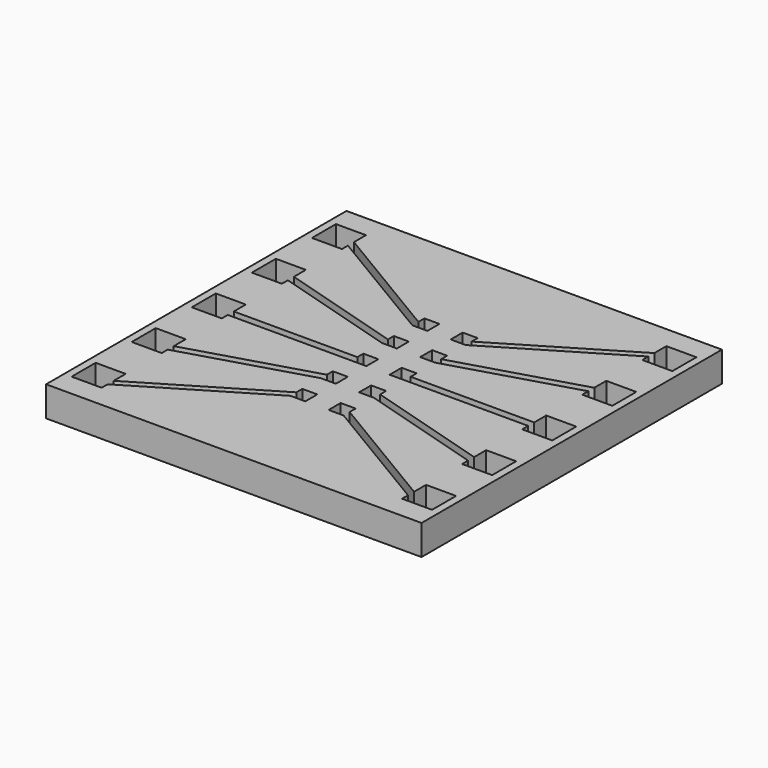
from build123d import *

# Parameters (mm, degrees)
F0_W     = 25
F0_H     = 25
F1_DEPTH = 2
F3_DEPTH = 2


# Not quite as in the source:
# - a feature names something its author has since deleted; it is built from what else it names


with BuildPart() as f1:
    # F0 (on Top) → F1 (new body)
    with BuildSketch(Plane.XY):
        with Locations((-12.5, 12.5)):
            Rectangle(F0_W, F0_H)
    extrude(amount=F1_DEPTH)

    # F2 (on face) → F3 (cut)
    with BuildSketch(Plane.XY.offset(2)):
        Polygon((-13.275, 15.54), (-14.275, 15.54), (-14.275, 15.04), (-22.5, 17.5), (-22.5, 18.5), (-24.5, 18.5), (-24.5, 16.5), (-22.5, 16.5), (-22.5, 17), (-14.275, 14.54), (-13.275, 14.54), align=None)
        Polygon((-13.275, 18.08), (-14.275, 18.08), (-14.275, 17.58), (-22.5, 22.5), (-22.5, 23.5), (-24.5, 23.5), (-24.5, 21.5), (-22.5, 21.5), (-22.5, 22), (-14.275, 17.08), (-13.275, 17.08), align=None)
        Polygon((-13.275, 13), (-14.275, 13), (-14.275, 12.5), (-22.5, 12.5), (-22.5, 13.5), (-24.5, 13.5), (-24.5, 11.5), (-22.5, 11.5), (-22.5, 12), (-14.275, 12), (-13.275, 12), align=None)
        Polygon((-13.275, 10.46), (-14.275, 10.46), (-14.275, 9.96), (-22.5, 7.5), (-22.5, 8.5), (-24.5, 8.5), (-24.5, 6.5), (-22.5, 6.5), (-22.5, 7), (-14.275, 9.46), (-13.275, 9.46), align=None)
        Polygon((-13.275, 7.92), (-14.275, 7.92), (-14.275, 7.42), (-22.5, 2.5), (-22.5, 3.5), (-24.5, 3.5), (-24.5, 1.5), (-22.5, 1.5), (-22.5, 2), (-14.275, 6.92), (-13.275, 6.92), align=None)
        Polygon((-10.725, 6.92), (-2.5, 2), (-2.5, 1.5), (-0.5, 1.5), (-0.5, 3.5), (-2.5, 3.5), (-2.5, 2.5), (-10.725, 7.42), (-10.725, 7.92), (-11.725, 7.92), (-11.725, 6.92), align=None)
        Polygon((-11.725, 12), (-10.725, 12), (-2.5, 12), (-2.5, 11.5), (-0.5, 11.5), (-0.5, 13.5), (-2.5, 13.5), (-2.5, 12.5), (-10.725, 12.5), (-10.725, 13), (-11.725, 13), align=None)
        Polygon((-11.725, 14.54), (-10.725, 14.54), (-2.5, 17), (-2.5, 16.5), (-0.5, 16.5), (-0.5, 18.5), (-2.5, 18.5), (-2.5, 17.5), (-10.725, 15.04), (-10.725, 15.54), (-11.725, 15.54), align=None)
        Polygon((-10.725, 17.58), (-10.725, 18.08), (-11.725, 18.08), (-11.725, 17.08), (-10.725, 17.08), (-2.5, 22), (-2.5, 21.5), (-0.5, 21.5), (-0.5, 23.5), (-2.5, 23.5), (-2.5, 22.5), align=None)
        Polygon((-10.725, 9.96), (-10.725, 10.46), (-11.725, 10.46), (-11.725, 9.46), (-10.725, 9.46), (-2.5, 7), (-2.5, 6.5), (-0.5, 6.5), (-0.5, 8.5), (-2.5, 8.5), (-2.5, 7.5), align=None)
    extrude(amount=-F3_DEPTH, mode=Mode.SUBTRACT)


solid = f1.part
